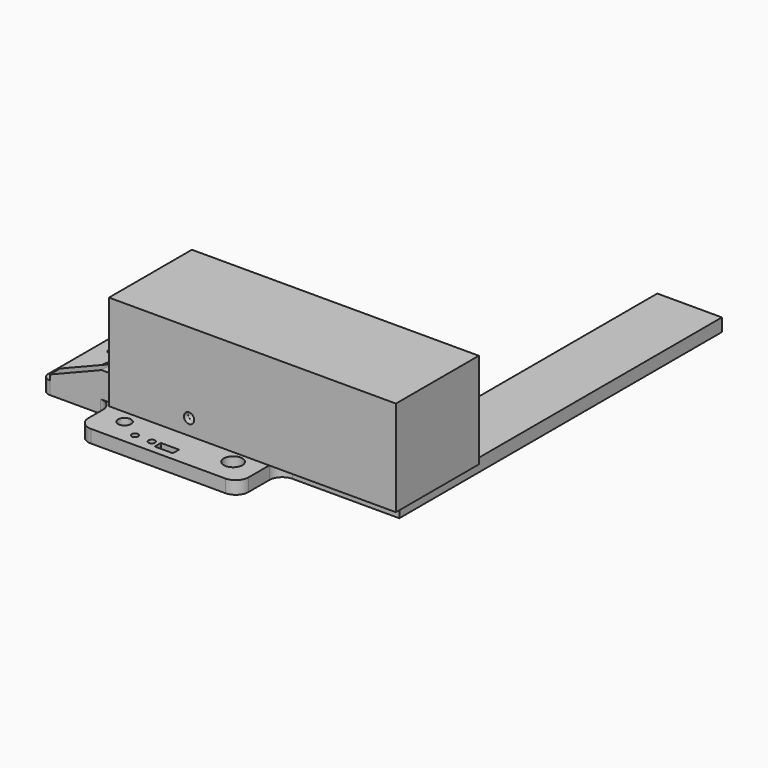
from build123d import *

# Parameters (mm, degrees)
F0_R        = 1.5
F0_R_2      = 6
F0_R_3      = 2.5
F0_R_4      = 1.25
F0_W        = 7
F0_H        = 3
F0_R_5      = 3.6
F0_R_6      = 1.75
F1_DEPTH    = 2.5
F2_R        = 5
F3_R        = 3
F6_DEPTH    = 10
F7_C1_SIZE2 = 20
F7_C1_SIZE  = 8
F7_C2_SIZE2 = 8
F7_C2_SIZE  = 20
F7_C3_SIZE2 = 20
F7_C3_SIZE  = 8
F7_C4_SIZE2 = 8
F7_C4_SIZE  = 20
F10_DEPTH   = 111
F11_W       = 36.0851921141
F11_H       = 35
F12_DEPTH   = 2
F13_W       = 24.924390018
F13_H       = 20
F14_DEPTH   = 2
F15_R       = 2
F16_DEPTH   = 55.0435960571


# Not quite as in the source:
# - two fillets or chamfers of one size are made in one step


with BuildPart() as f1:
    # F0 (on Top) → F1 (new body, symmetric)
    with BuildSketch(Plane.XY):
        Polygon((66.28, 141), (66.28, 35), (-16.99, 35), (-16.99, 18), (-44.52, 18), (-44.52, -18), (-16.99, -18), (-16.99, -35), (45, -35), (45, -15), (91.28, -15), (91.28, 141), align=None)
        with Locations((-38.52, -8.5)):
            Circle(F0_R, mode=Mode.SUBTRACT)
        with Locations((-38.52, 8.5)):
            Circle(F0_R, mode=Mode.SUBTRACT)
        with Locations((-29.52, 0)):
            Circle(F0_R_2, mode=Mode.SUBTRACT)
        with Locations((-26.52, -8.5)):
            Circle(F0_R, mode=Mode.SUBTRACT)
        with Locations((-26.52, 8.5)):
            Circle(F0_R, mode=Mode.SUBTRACT)
        with Locations((-6.99, -25)):
            Circle(F0_R_3, mode=Mode.SUBTRACT)
        with Locations((1.04, -30)):
            Circle(F0_R_4, mode=Mode.SUBTRACT)
        with Locations((7.54, -30)):
            Circle(F0_R_4, mode=Mode.SUBTRACT)
        with Locations((13.78, -30.5)):
            Rectangle(F0_W, F0_H, mode=Mode.SUBTRACT)
        with Locations((-6.99, 25)):
            Circle(F0_R_3, mode=Mode.SUBTRACT)
        with Locations((1.04, 30)):
            Circle(F0_R_4, mode=Mode.SUBTRACT)
        with Locations((7.54, 30)):
            Circle(F0_R_4, mode=Mode.SUBTRACT)
        with Locations((13.78, 30.5)):
            Rectangle(F0_W, F0_H, mode=Mode.SUBTRACT)
        with Locations((35, -25)):
            Circle(F0_R_5, mode=Mode.SUBTRACT)
        with Locations((78.78, -5)):
            Circle(F0_R_6, mode=Mode.SUBTRACT)
        with Locations((78.78, 5)):
            Circle(F0_R_6, mode=Mode.SUBTRACT)
        with Locations((35, 25)):
            Circle(F0_R_5, mode=Mode.SUBTRACT)
    extrude(amount=F1_DEPTH, both=True)

    # F2
    f2_edges = [f1.edges().sort_by_distance(p)[0] for p in [
        (-16.99, -35, 0),
        (66.28, 35, 0),
        (45, -15, 0),
        (45, -35, 0),
        (-16.99, -18, 0),
        (-16.99, 18, 0),
        (-16.99, 35, 0),
    ]]
    fillet(f2_edges, radius=F2_R)

    # F3
    f3_edges = [f1.edges().sort_by_distance(p)[0] for p in [
        (-44.52, -18, 0),
        (-44.52, 18, 0),
    ]]
    fillet(f3_edges, radius=F3_R)

    # F5 (on face) → F6 (join)
    with BuildSketch(Plane.XY.offset(2.5)):
        Polygon((-21.99, 18), (-41.52, 18), (-41.52, 13), (62.2002519667, 13), (62.2002519667, 18), align=None)
        Polygon((-41.52, -13), (-41.52, -18), (-21.99, -18), (43.2625375688, -18), (43.2625375688, -13), align=None)
    extrude(amount=F6_DEPTH)

    # F7: chamfer of 8 x 20 on 4 edges, made by hand

    # F7_c1
    f7_c1_edges = [f1.edges().sort_by_distance(p)[0] for p in [
        (62.2002519667, 15.5, 12.5),
    ]]
    f7_c1_side = f1.faces().sort_by_distance((62.2002519667, 15.5, 12.34))[0]
    chamfer(f7_c1_edges, length=F7_C1_SIZE, length2=F7_C1_SIZE2, reference=f7_c1_side)

    # F7_c2
    f7_c2_edges = [f1.edges().sort_by_distance(p)[0] for p in [
        (-41.52, 15.5, 12.5),
    ]]
    f7_c2_side = f1.faces().sort_by_distance((-41.36, 15.5, 12.5))[0]
    chamfer(f7_c2_edges, length=F7_C2_SIZE, length2=F7_C2_SIZE2, reference=f7_c2_side)

    # F7_c3
    f7_c3_edges = [f1.edges().sort_by_distance(p)[0] for p in [
        (43.2625375688, -15.5, 12.5),
    ]]
    f7_c3_side = f1.faces().sort_by_distance((43.2625375688, -15.5, 12.34))[0]
    chamfer(f7_c3_edges, length=F7_C3_SIZE, length2=F7_C3_SIZE2, reference=f7_c3_side)

    # F7_c4
    f7_c4_edges = [f1.edges().sort_by_distance(p)[0] for p in [
        (-41.52, -15.5, 12.5),
    ]]
    f7_c4_side = f1.faces().sort_by_distance((-41.36, -15.5, 12.5))[0]
    chamfer(f7_c4_edges, length=F7_C4_SIZE, length2=F7_C4_SIZE2, reference=f7_c4_side)


with BuildPart() as f10:
    # F9 (on face) → F10 (new body)
    with BuildSketch(Plane(origin=(-16.99, 0, 0), x_dir=(0, -1, 0), z_dir=(-1, 0, 0))):
        Polygon((-20.0425960571, 2.5), (-18.0425960571, 2.5), (-18.0425960571, 37.5), (18.0425960571, 37.5), (18.0425960571, 2.5), (20.0425960571, 2.5), (20.0425960571, 39.5), (-20.0425960571, 39.5), align=None)
    extrude(amount=-F10_DEPTH)

    # F11 (on face) → F12 (join)
    with BuildSketch(Plane.YZ.offset(94.01)):
        with Locations((0, 20)):
            Rectangle(F11_W, F11_H)
    extrude(amount=-F12_DEPTH)

    # F13 (on face) → F14 (cut)
    with BuildSketch(Plane(origin=(0, 20.0425960571, 0), x_dir=(-1, 0, 0), z_dir=(0, 1, 0))):
        with Locations((-78.9941735566, 12.5)):
            Rectangle(F13_W, F13_H)
    extrude(amount=-F14_DEPTH, mode=Mode.SUBTRACT)


with BuildPart() as f16_tool:
    # F15 (on face) → F16 (new body, through all)
    with BuildSketch(Plane(origin=(0, 20.0425960571, 0), x_dir=(-1, 0, 0), z_dir=(0, 1, 0))):
        with Locations((-13.9942942187, 8.5)):
            Circle(F15_R)
    extrude(amount=-F16_DEPTH)


with BuildPart() as f1_1:
    add(f1.part)

    # F16: cut by f16_tool
    add(f16_tool.part, mode=Mode.SUBTRACT)


with BuildPart() as f10_1:
    add(f10.part)

    # F16: cut by f16_tool
    add(f16_tool.part, mode=Mode.SUBTRACT)


solid = Compound([f1_1.part, f10_1.part])
